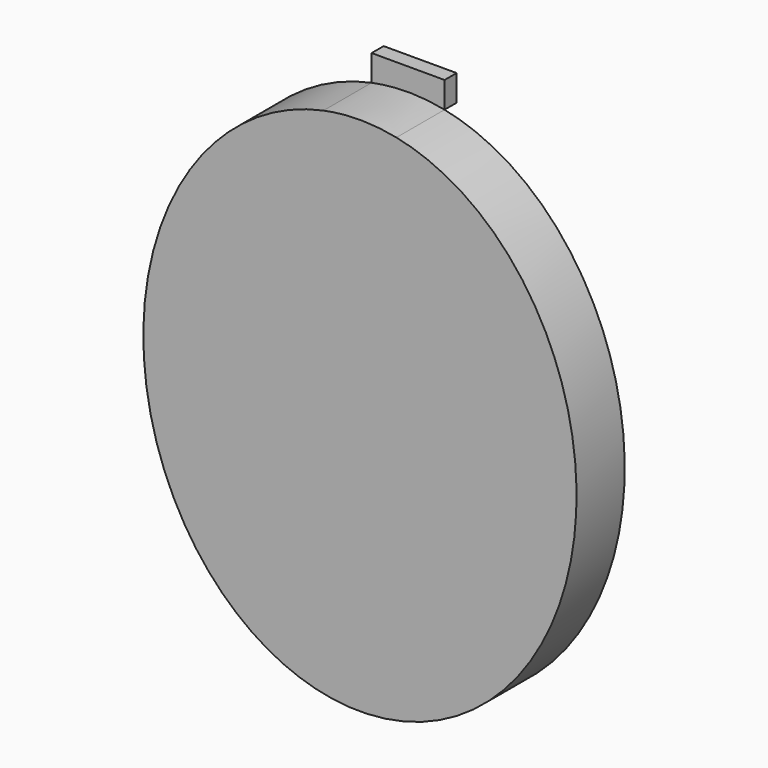
from build123d import *

# Parameters (mm, degrees)
F0_W     = 15.3937507421
F0_H     = 6.1911940575
F1_DEPTH = 12.7
F2_DEPTH = 3.175


# Not quite as in the source:
# - a feature names something its author has since deleted; it is built from what else it names


with BuildPart() as f1:
    # F0 (on Front) → F1 (new body)
    with BuildSketch(Plane.XZ):
        with BuildLine():
            Line((-7.696875371, 50.2006262541), (-7.696875371, 54.1549392845))
            add(Edge.make_bspline(
                [(-7.696875371, 54.1549392845), (-76.4624997725, 40.0336773305), (-38.2312498863, -30.1082268122), (0, -100.2501309548), (38.2312498863, -30.1082268122), (76.4624997725, 40.0336773305), (7.696875371, 54.1549392845)],
                knots=[0.16920633, 0.16920633, 0.16920633, 2.1507972124, 2.1507972124, 4.1323880948, 4.1323880948, 6.1139789772, 6.1139789772, 6.1139789772], degree=2, weights=[1, 0.5480246776, 1, 0.5480246776, 1, 0.5480246776, 1]))
            Line((7.696875371, 54.1549392845), (7.696875371, 50.2006262541))
            Line((7.696875371, 50.2006262541), (7.696875371, 44.0094321966))
            Line((7.696875371, 44.0094321966), (-7.696875371, 44.0094321966))
            Line((-7.696875371, 44.0094321966), (-7.696875371, 50.2006262541))
        make_face()
        with BuildLine():
            add(Edge.make_bspline(
                [(7.696875371, 54.1549392845), (3.8761156095, 54.939545691), (0, 54.939545691)],
                knots=[6.1139789772, 6.1139789772, 6.1139789772, 6.2831853072, 6.2831853072, 6.2831853072], degree=2, weights=[1, 0.9964232864, 1]))
            add(Edge.make_bspline(
                [(0, 54.939545691), (-3.8761156095, 54.939545691), (-7.696875371, 54.1549392845)],
                knots=[0, 0, 0, 0.16920633, 0.16920633, 0.16920633], degree=2, weights=[1, 0.9964232864, 1]))
            Line((-7.696875371, 54.1549392845), (-7.696875371, 50.2006262541))
            Line((-7.696875371, 50.2006262541), (7.696875371, 50.2006262541))
            Line((7.696875371, 50.2006262541), (7.696875371, 54.1549392845))
        make_face()
        with Locations((0, 47.1050292253)):
            Rectangle(F0_W, F0_H)
    extrude(amount=F1_DEPTH)


with BuildPart() as f2:
    # F0 (on Front) → F2 (new body)
    with BuildSketch(Plane.XZ):
        with BuildLine():
            add(Edge.make_bspline(
                [(0, 54.939545691), (-3.8761156095, 54.939545691), (-7.696875371, 54.1549392845)],
                knots=[0, 0, 0, 0.16920633, 0.16920633, 0.16920633], degree=2, weights=[1, 0.9964232864, 1]))
            add(Edge.make_bspline(
                [(7.696875371, 54.1549392845), (3.8761156095, 54.939545691), (0, 54.939545691)],
                knots=[6.1139789772, 6.1139789772, 6.1139789772, 6.2831853072, 6.2831853072, 6.2831853072], degree=2, weights=[1, 0.9964232864, 1]))
            Line((7.696875371, 54.1549392845), (7.696875371, 59.6784651279))
            Line((7.696875371, 59.6784651279), (-7.696875371, 59.6784651279))
            Line((-7.696875371, 59.6784651279), (-7.696875371, 54.1549392845))
        make_face()
    extrude(amount=-F2_DEPTH)


solid = Compound([f1.part, f2.part])
